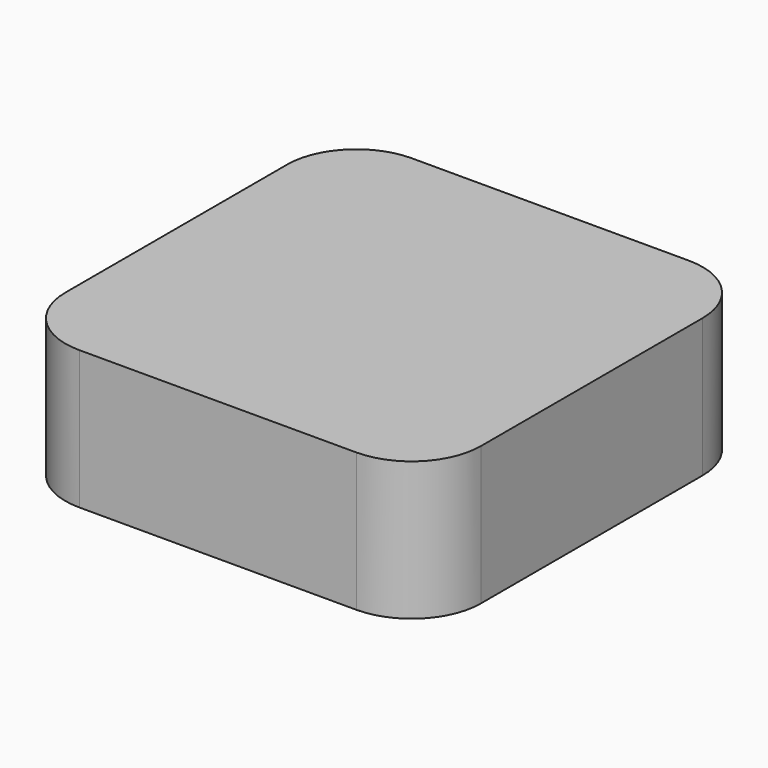
from build123d import *

# Parameters (mm, degrees)
F0_W          = 4.7625
F0_H          = 4.7625
F1_DEPTH      = 3.175
F2_R          = 0.396875
F5_DEPTH      = 6.35
F5_DEPTH_BACK = 6.35


# Not quite as in the source:
# - a length typed as a fraction of an inch, garbled in the dataset ("3 / 203.2 mm" for 3/8 in), is restored


with BuildPart() as f1:
    # F0 (on Top) → F1 (new body)
    with BuildSketch(Plane.XY):
        with BuildLine():
            ThreePointArc((2.38125, 6.35), (2.1487660076, 6.9112660076), (1.5875, 7.14375))
            Line((1.5875, 7.14375), (-1.5875, 7.14375))
            ThreePointArc((-1.5875, 7.14375), (-2.1487660076, 6.9112660076), (-2.38125, 6.35))
            Line((-2.38125, 6.35), (-2.38125, 2.38125))
            Line((-2.38125, 2.38125), (2.38125, 2.38125))
            Line((2.38125, 2.38125), (2.38125, 6.35))
        make_face()
        with BuildLine():
            Line((6.35, 2.38125), (2.38125, 2.38125))
            Line((2.38125, 2.38125), (2.38125, -2.38125))
            Line((2.38125, -2.38125), (6.35, -2.38125))
            ThreePointArc((6.35, -2.38125), (6.9112660076, -2.1487660076), (7.14375, -1.5875))
            Line((7.14375, -1.5875), (7.14375, 1.5875))
            ThreePointArc((7.14375, 1.5875), (6.9112660076, 2.1487660076), (6.35, 2.38125))
        make_face()
        Rectangle(F0_W, F0_H)
        with BuildLine():
            Line((-2.38125, -2.38125), (-2.38125, 2.38125))
            Line((-2.38125, 2.38125), (-6.35, 2.38125))
            ThreePointArc((-6.35, 2.38125), (-6.9112660076, 2.1487660076), (-7.14375, 1.5875))
            Line((-7.14375, 1.5875), (-7.14375, -1.5875))
            ThreePointArc((-7.14375, -1.5875), (-6.9112660076, -2.1487660076), (-6.35, -2.38125))
            Line((-6.35, -2.38125), (-2.38125, -2.38125))
        make_face()
        with BuildLine():
            Line((2.38125, -6.35), (2.38125, -2.38125))
            Line((2.38125, -2.38125), (-2.38125, -2.38125))
            Line((-2.38125, -2.38125), (-2.38125, -6.35))
            ThreePointArc((-2.38125, -6.35), (-2.1487660076, -6.9112660076), (-1.5875, -7.14375))
            Line((-1.5875, -7.14375), (1.5875, -7.14375))
            ThreePointArc((1.5875, -7.14375), (2.1487660076, -6.9112660076), (2.38125, -6.35))
        make_face()
    extrude(amount=F1_DEPTH)

    # F2
    f2_edges = [f1.edges().sort_by_distance(p)[0] for p in [
        (2.38125, 4.365625, 3.175),
        (2.148766, 6.911266, 3.175),
        (0, 7.14375, 3.175),
        (-2.148766, 6.911266, 3.175),
        (-2.38125, 4.365625, 3.175),
        (-4.365625, 2.38125, 3.175),
        (-6.911266, 2.148766, 3.175),
        (-7.14375, 0, 3.175),
        (-6.911266, -2.148766, 3.175),
        (-4.365625, -2.38125, 3.175),
        (-2.38125, -4.365625, 3.175),
        (-2.148766, -6.911266, 3.175),
        (0, -7.14375, 3.175),
        (2.148766, -6.911266, 3.175),
        (2.38125, -4.365625, 3.175),
        (4.365625, -2.38125, 3.175),
        (6.911266, -2.148766, 3.175),
        (7.14375, 0, 3.175),
        (6.911266, 2.148766, 3.175),
        (4.365625, 2.38125, 3.175),
        (2.38125, 4.365625, 0),
        (2.148766, 6.911266, 0),
        (0, 7.14375, 0),
        (-2.148766, 6.911266, 0),
        (-2.38125, 4.365625, 0),
        (-4.365625, 2.38125, 0),
        (-6.911266, 2.148766, 0),
        (-7.14375, 0, 0),
        (-6.911266, -2.148766, 0),
        (-4.365625, -2.38125, 0),
        (-2.38125, -4.365625, 0),
        (-2.148766, -6.911266, 0),
        (0, -7.14375, 0),
        (2.148766, -6.911266, 0),
        (2.38125, -4.365625, 0),
        (4.365625, -2.38125, 0),
        (6.911266, -2.148766, 0),
        (7.14375, 0, 0),
        (6.911266, 2.148766, 0),
        (4.365625, 2.38125, 0),
    ]]
    fillet(f2_edges, radius=F2_R)


with BuildPart() as f5:
    # F4 (on offset) → F5 (new body, two sides)
    with BuildSketch(Plane.XY.offset(1.5875)) as f5_sk:
        with BuildLine():
            ThreePointArc((19.05, 12.7), (17.1901280605, 17.1901280605), (12.7, 19.05))
            Line((12.7, 19.05), (-12.7, 19.05))
            ThreePointArc((-12.7, 19.05), (-17.1901280605, 17.1901280605), (-19.05, 12.7))
            Line((-19.05, 12.7), (-19.05, -12.7))
            ThreePointArc((-19.05, -12.7), (-17.1901280605, -17.1901280605), (-12.7, -19.05))
            Line((-12.7, -19.05), (12.7, -19.05))
            ThreePointArc((12.7, -19.05), (17.1901280605, -17.1901280605), (19.05, -12.7))
            Line((19.05, -12.7), (19.05, 12.7))
        make_face()
    extrude(amount=F5_DEPTH)
    extrude(f5_sk.sketch, amount=-F5_DEPTH_BACK)


solid = Compound([f1.part, f5.part])
